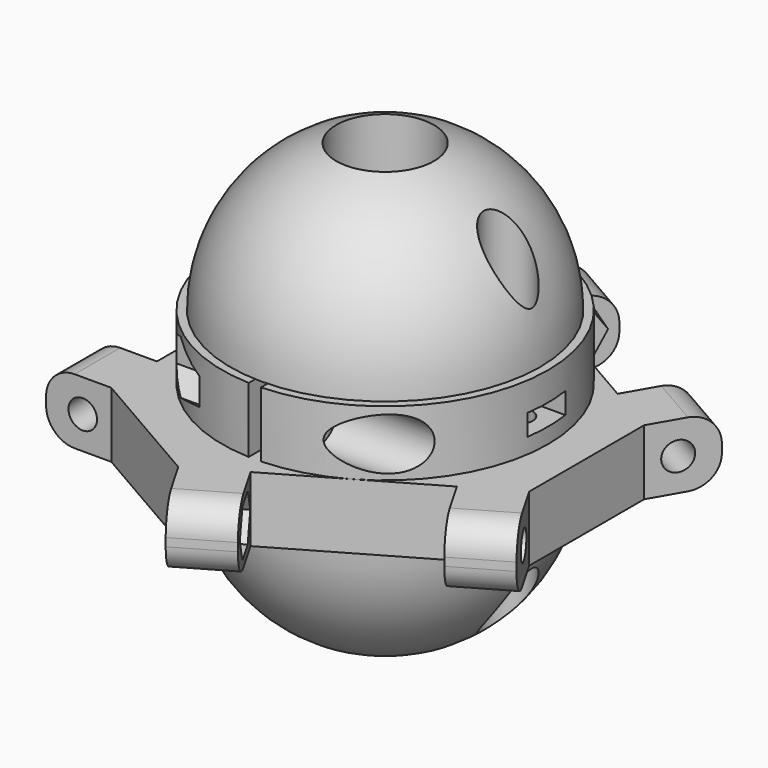
from build123d import *

# Parameters (mm, degrees)
F1_DEPTH         = 8
F3_R             = 8
F4_DEPTH         = 3
F5_R             = 1.75
F6_DEPTH         = 13.8602177134
F9_END_RADIUS    = 20
F8_R             = 3.2
F9_REACH         = 25.0519668992
F11_DEPTH        = 8
F13_W            = 5.8
F13_H            = 2.6
F14_REACH        = 14.8570995328
F16_ANGLE        = 180
F17_R            = 10.5
F18_DEPTH        = 8
F19_R            = 3.5
F21_ANGLE        = 30
F22_R            = 1.75
F23_DEPTH        = 57.6240669589
F23_COPIES_COUNT = 3
F26_DEPTH        = 25
F26_COPIES_COUNT = 3
F28_D            = 3.5
F28_CBORE_D      = 5.9
F28_CBORE_DEPTH  = 3.2
F32_R            = 4
F33_DEPTH        = 34.0287563773
F35_R            = 1.75
F36_DEPTH        = 19.0010001
F37_R            = 2.95
F38_DEPTH        = 25


# Not quite as in the source:
# - a pattern or mirror of a feature is missing from the dataset's text; its kind, count and spacing are read off the source's solid


with BuildPart() as f1:
    # F0 (on Top) → F1 (new body)
    with BuildSketch(Plane.XY):
        with BuildLine():
            Line((0.75, -6.0537178659), (0.75, -19.9859325527))
            ThreePointArc((0.75, -19.9859325527), (20, 0), (0.75, 19.9859325527))
            Line((0.75, 19.9859325527), (0.75, 6.0537178659))
            ThreePointArc((0.75, 6.0537178659), (6.1, 0), (0.75, -6.0537178659))
        make_face()
    extrude(amount=F1_DEPTH)

    # F3 (on face) → F4 (cut, through all)
    with BuildSketch(Plane.XY.offset(8)):
        Circle(F3_R)
    extrude(amount=-F4_DEPTH, mode=Mode.SUBTRACT)

    # F5 (on face) → F6 (cut, through all)
    with BuildSketch(Plane(origin=(0.75, 0, 0), x_dir=(0, -1, 0), z_dir=(-1, 0, 0))):
        with Locations((-15.4090907723, 3.9244145155)):
            Circle(F5_R)
        with Locations((15.4090907723, 3.9244145155)):
            Circle(F5_R)
    extrude(amount=-F6_DEPTH, mode=Mode.SUBTRACT)

    f9_end = (Plane(origin=(0, 0, 4), x_dir=(-1, 0, 0), z_dir=(0, 0, -1)) * Cylinder(F9_END_RADIUS, 140.2662879577, mode=Mode.PRIVATE)).faces().sort_by_distance((20, 0, 4))[0]
    # F8 (on offset) → F9 (cut, up to the whole of a round face its end follows)
    with BuildSketch(Plane.YZ.offset(4)):
        Polygon((12.5512069398, 5.5744145155), (12.5512069398, 2.2744145155), (15.4090907723, 0.6244145155), (18.2669746048, 2.2744145155), (18.2669746048, 5.5744145155), (15.4090907723, 7.2244145155), align=None)
        with Locations((-15.4090907722, 3.9244145155)):
            Circle(F8_R)
    f9_long = extrude(amount=F9_REACH, mode=Mode.PRIVATE)
    add(split(f9_long, bisect_by=f9_end, keep=Keep.BOTTOM, mode=Mode.PRIVATE), mode=Mode.SUBTRACT)

    # F10 (on face) → F11 (cut, through all)
    with BuildSketch(Plane.XY.offset(8)):
        with BuildLine():
            ThreePointArc((16.5, -1.6), (18.1, 0), (16.5, 1.6))
            Line((16.5, 1.6), (13.5, 1.6))
            ThreePointArc((13.5, 1.6), (11.9, 0), (13.5, -1.6))
            Line((13.5, -1.6), (16.5, -1.6))
        make_face()
    extrude(amount=-F11_DEPTH, mode=Mode.SUBTRACT)

    f14_end = f1.faces().sort_by_distance((20, 0, 4))[0]
    # F13 (on offset) → F14 (cut, up to a face of the model that its end follows)
    with BuildSketch(Plane.YZ.offset(11.5)):
        with Locations((0, 3.2)):
            Rectangle(F13_W, F13_H)
    f14_long = extrude(amount=F14_REACH, mode=Mode.PRIVATE)
    add(split(f14_long, bisect_by=f14_end, keep=Keep.BOTTOM, mode=Mode.PRIVATE), mode=Mode.SUBTRACT)


with BuildPart() as f16_1:
    # F16: copy of F1
    add(f1.part.rotate(Axis((0, 0, 10.0987032056), (0, 0, 1)), F16_ANGLE))


with BuildPart() as f18:
    # F17 (on face) → F18 (new body)
    with BuildSketch(Plane(origin=(0, 0, 0), x_dir=(1, 0, 0), z_dir=(0, 0, -1))):
        Polygon((25.8205080757, 4.7224318643), (17, 20), (17, 28), (10, 28), (10, 20), (-10, 20), (-10, 28), (-17, 28), (-17, 20), (-25.8205080757, 4.7224318643), (-32.748711306, 0.7224318643), (-29.248711306, -5.3397459622), (-22.3205080757, -1.3397459622), (-12.3205080757, -18.6602540378), (-19.248711306, -22.6602540378), (-15.748711306, -28.7224318643), (-8.8205080757, -24.7224318643), (8.8205080757, -24.7224318643), (15.748711306, -28.7224318643), (19.248711306, -22.6602540378), (12.3205080757, -18.6602540378), (22.3205080757, -1.3397459622), (29.248711306, -5.3397459622), (32.748711306, 0.7224318643), align=None)
        Circle(F17_R, mode=Mode.SUBTRACT)
    extrude(amount=F18_DEPTH)

    # F19
    f19_edges = [f18.edges().sort_by_distance(p)[0] for p in [
        (30.998711, 2.308657, -8),
        (30.998711, 2.308657, 0),
        (17.498711, 25.691343, -8),
        (17.498711, 25.691343, 0),
        (-17.498711, 25.691343, -8),
        (-17.498711, 25.691343, 0),
        (-30.998711, 2.308657, -8),
        (-30.998711, 2.308657, 0),
        (-13.5, -28, -8),
        (13.5, -28, -8),
        (-13.5, -28, 0),
        (13.5, -28, 0),
    ]]
    fillet(f19_edges, radius=F19_R)


with BuildPart() as f18_1:
    # F21: moved
    add(f18.part.rotate(Axis((0, 0, 17.0708075166), (0, 0, 1)), F21_ANGLE))

    # F22 (on face) → F23 (cut, through all)
    with BuildSketch(Plane(origin=(14.7224318643, 8.5, 0), x_dir=(-0.5, 0.8660254038, 0), z_dir=(0.8660254038, 0.5, 0))):
        with Locations((-23.5, -4)):
            Circle(F22_R)
    f23 = extrude(amount=-F23_DEPTH, mode=Mode.SUBTRACT)

    # F23_copies: F23 ×3 about axis
    f23_copies_axis = Axis((0, 0, 0), (0, 0, 1))
    for i in range(1, F23_COPIES_COUNT):
        add(f23.rotate(f23_copies_axis, i * 360 / F23_COPIES_COUNT), mode=Mode.SUBTRACT)

    # F25 (on offset) → F26 (cut)
    with BuildSketch(Plane(origin=(11.6913429511, 6.75, 0), x_dir=(0.5, -0.8660254038, 0), z_dir=(-0.8660254038, -0.5, 0))):
        Polygon((25.164795125, -6.9000154874), (26.8391109057, -4.0000154874), (25.164795125, -1.1000154874), (21.8161635637, -1.1000154874), (20.1418477831, -4.0000154874), (21.8161635637, -6.9000154874), align=None)
    f26 = extrude(amount=F26_DEPTH, mode=Mode.SUBTRACT)

    # F26_copies: F26 ×3 about axis
    f26_copies_axis = Axis((0, 0, 0), (0, 0, 1))
    for i in range(1, F26_COPIES_COUNT):
        add(f26.rotate(f26_copies_axis, i * 360 / F26_COPIES_COUNT), mode=Mode.SUBTRACT)

    # F28 (through all)
    with Locations(Plane(origin=(0, 0, -8), x_dir=(1, 0, 0), z_dir=(0, 0, -1))):
        with Locations((15.0597468019, 0), (-15.0597468019, 0)):
            CounterBoreHole(F28_D / 2, F28_CBORE_D / 2, F28_CBORE_DEPTH)


with BuildPart() as f31:
    # F30 (on line) → F31 (revolve)
    with BuildSketch(Plane.YZ):
        with BuildLine():
            Line((-6, -8), (-19, -8))
            ThreePointArc((-19, -8), (-15.4110350074, -19.1130553854), (-6, -26.0277563773))
            Line((-6, -26.0277563773), (-6, -8))
        make_face()
    revolve(axis=Axis((0, 0, 17.0708075166), (0, 0, 1)))

    # F35 (on offset) → F36 (cut, through all)
    with BuildSketch(Plane(origin=(0, 0, -11), x_dir=(1, 0, 0), z_dir=(0, 0, -1))):
        with Locations((-15.0597468019, 0)):
            Circle(F35_R)
        with Locations((15.0597468019, 0)):
            Circle(F35_R)
    extrude(amount=-F36_DEPTH, mode=Mode.SUBTRACT)

    # F37 (on offset) → F38 (cut)
    with BuildSketch(Plane(origin=(0, 0, -11), x_dir=(1, 0, 0), z_dir=(0, 0, -1))):
        with Locations((-15.0597468019, 0)):
            Circle(F37_R)
        with Locations((15.0597468019, 0)):
            Circle(F37_R)
    extrude(amount=F38_DEPTH, mode=Mode.SUBTRACT)


with BuildPart() as f33_tool:
    # F32 (on face) → F33 (new body, through all)
    with BuildSketch(Plane.XY.offset(8)):
        with Locations((0, 9.2912273748)):
            Circle(F32_R)
        with Locations((0, -9.2912273748)):
            Circle(F32_R)
    extrude(amount=-F33_DEPTH)


with BuildPart() as f1_1:
    add(f1.part)

    # F33: cut by f33_tool
    add(f33_tool.part, mode=Mode.SUBTRACT)


with BuildPart() as f16_1_1:
    add(f16_1.part)

    # F33: cut by f33_tool
    add(f33_tool.part, mode=Mode.SUBTRACT)


with BuildPart() as f18_2:
    add(f18_1.part)

    # F33: cut by f33_tool
    add(f33_tool.part, mode=Mode.SUBTRACT)


with BuildPart() as f39_1:
    # F39: instance of F31
    add(f31.part.mirror(Plane.XY))


solid = Compound([f31.part, f1_1.part, f16_1_1.part, f18_2.part, f39_1.part])
